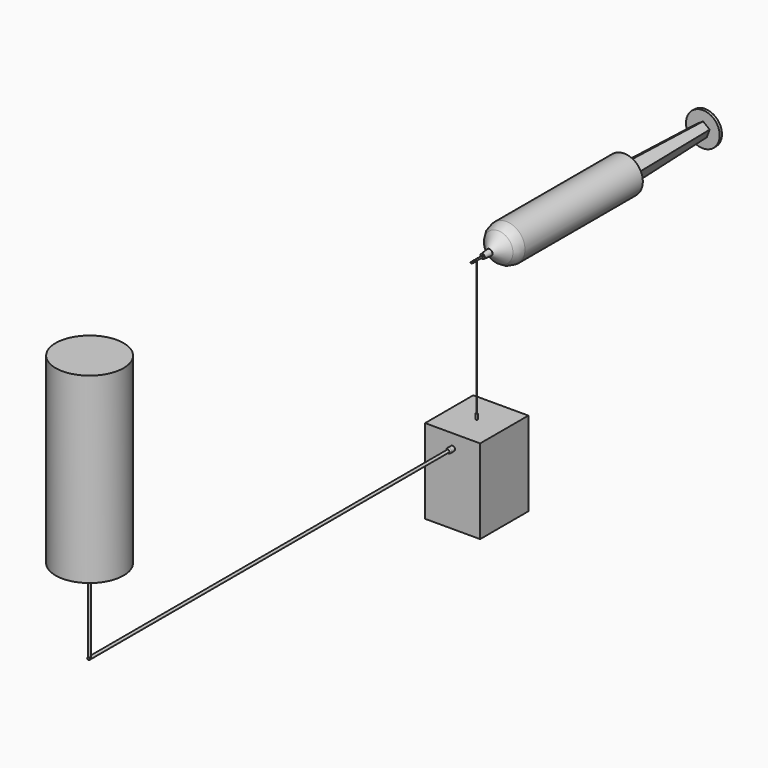
from build123d import *

# Parameters (mm, degrees)
F0_R         = 6.635
F1_DEPTH     = 60
F2_R         = 5.5640936577
F3_DEPTH     = 55
F5_DEPTH     = 90
F5_TAPER     = 1.5
F6_R         = 6
F7_DEPTH     = 1
F8_SIZE      = 5.5
F9_R         = 5
F10_R        = 1.1188654797
F11_DEPTH    = 3
F11_TAPER    = 6
F12_R        = 0.2661166515
F13_DEPTH    = 5
F15_START    = -0.7
F14_R        = 0.3090418991
F14_R_2      = 0.2661166515
F15_DEPTH    = 0.76
F17_START    = -2
F16_R        = 0.3072145748
F17_DEPTH    = 0.79
F19_R        = 0.1295808952
F20_DEPTH    = 50
F21_W        = 19.5904374123
F21_H        = 21.4598029852
F22_DEPTH    = 30
F23_R        = 0.3370193149
F24_DEPTH    = 2
F25_R        = 0.3
F26_R        = 0.8572593425
F27_DEPTH    = 2
F28_R        = 0.4
F29_R        = 1.2929704819
F29_R_2      = 1.8897224416
F29_R_3      = 1.1340105919
F30_DEPTH    = 1
F31_R        = 0.4652474762
F32_DEPTH    = 160
F35_R        = 0.4356898576
F36_DEPTH    = 30
F37_F1_R     = 0.02
F37_F2_R     = 0.02
F37_T6_ANGLE = 55.0572993012
F37_S7_R     = 0.4652474762
F37_T8_DEPTH = 2
F38_R        = 12.0941748202
F39_DEPTH    = 65


# Not quite as in the source:
# - a fillet or chamfer that OpenCascade refuses, or shapes differently, is made with other operations: its cross-section is extruded or revolved along the edge and cut away or added
# - a feature of the source that left no trace in its solid (it failed there, or was rolled back) is left out


with BuildPart() as f1:
    # F0 (on Front) → F1 (new body)
    with BuildSketch(Plane.XZ):
        Circle(F0_R)
    extrude(amount=F1_DEPTH)

    # F2 (on face) → F3 (cut)
    with BuildSketch(Plane(origin=(0, 0, 0), x_dir=(-1, 0, 0), z_dir=(0, 1, 0))):
        Circle(F2_R)
    extrude(amount=-F3_DEPTH, mode=Mode.SUBTRACT)

    # F4 (on face) → F5 (join)
    with BuildSketch(Plane(origin=(0, -55, 0), x_dir=(-1, 0, 0), z_dir=(0, 1, 0))):
        Polygon((-0.2330018257, 5.4173569127), (-5.2242141168, 1.452457446), (-2.995740063, -4.5196888438), (3.3727449364, -4.24577877), (5.080211069, 1.8956532552), align=None)
    extrude(amount=F5_DEPTH, taper=F5_TAPER)

    # F6 (on face) → F7 (join)
    with BuildSketch(Plane(origin=(0, 35, 0), x_dir=(-1, 0, 0), z_dir=(0, 1, 0))):
        Circle(F6_R)
    extrude(amount=F7_DEPTH)

    # F8
    f8_edges = [f1.edges().sort_by_distance(p)[0] for p in [
        (-6.635, -60, 0),
    ]]
    chamfer(f8_edges, length=F8_SIZE)

    # F9
    f9_edges = [f1.edges().sort_by_distance(p)[0] for p in [
        (-6.635, -54.5, 0),
    ]]
    fillet(f9_edges, radius=F9_R)

    # F10 (on face) → F11 (join)
    with BuildSketch(Plane.XZ.offset(60)):
        Circle(F10_R)
    extrude(amount=F11_DEPTH, taper=F11_TAPER)


with BuildPart() as f13:
    # F12 (on face) → F13 (new body)
    with BuildSketch(Plane.XZ.offset(63)):
        Circle(F12_R)
    extrude(amount=F13_DEPTH)


with BuildPart() as f15:
    # F14 (on face) → F15 (new body)
    with BuildSketch(Plane.XZ.offset(68).offset(F15_START)):
        Circle(F14_R)
        Circle(F14_R_2, mode=Mode.SUBTRACT)
    extrude(amount=-F15_DEPTH)


with BuildPart() as f17:
    # F16 (on face) → F17 (new body)
    with BuildSketch(Plane.XZ.offset(68).offset(F17_START)):
        Circle(F16_R)
    extrude(amount=-F17_DEPTH)


with BuildPart() as f20:
    # F19 (on Top) → F20 (new body)
    with BuildSketch(Plane.XY):
        with Locations((0, -65.6076744199)):
            Circle(F19_R)
    extrude(amount=-F20_DEPTH)


with BuildPart() as f22:
    # F21 (on face) → F22 (new body)
    with BuildSketch(Plane(origin=(0, 0, -50), x_dir=(1, 0, 0), z_dir=(0, 0, -1))):
        with Locations((0, 65.6076744199)):
            Rectangle(F21_W, F21_H)
    extrude(amount=F22_DEPTH)

    # F29 (on face) → F30 (cut)
    with BuildSketch(Plane(origin=(-9.7952187061, 0, 0), x_dir=(0, -1, 0), z_dir=(-1, 0, 0))):
        with Locations((59.0209439397, -53.7652634084)):
            Circle(F29_R)
        with Locations((59.1616034508, -58.758571744)):
            Circle(F29_R_2)
        with Locations((59.3022592366, -63.3299127221)):
            Circle(F29_R_3)
    extrude(amount=-F30_DEPTH, mode=Mode.SUBTRACT)


with BuildPart() as f24:
    # F23 (on face) → F24 (new body)
    with BuildSketch(Plane.XY.offset(-50)):
        with Locations((0, -65.6058713794)):
            Circle(F23_R)
    extrude(amount=F24_DEPTH)

    # F25
    f25_edges = [f24.edges().sort_by_distance(p)[0] for p in [
        (-0.337019, -65.605871, -48),
    ]]
    fillet(f25_edges, radius=F25_R)


with BuildPart() as f27:
    # F26 (on face) → F27 (new body)
    with BuildSketch(Plane.XZ.offset(76.3375759125)):
        with Locations((0, -54.7743812203)):
            Circle(F26_R)
    extrude(amount=F27_DEPTH)

    # F28
    f28_edges = [f27.edges().sort_by_distance(p)[0] for p in [
        (-0.857259, -78.337576, -54.774381),
    ]]
    fillet(f28_edges, radius=F28_R)


with BuildPart() as f32:
    # F31 (on face) → F32 (new body)
    with BuildSketch(Plane.XZ.offset(78.3375759125)):
        with Locations((0, -54.7743812203)):
            Circle(F31_R)
    extrude(amount=F32_DEPTH)

    # F35 (on offset) → F36 (join)
    with BuildSketch(Plane.XY.offset(-55)):
        with Locations((0, -237.8518730402)):
            Circle(F35_R)
    extrude(amount=F36_DEPTH)

    # F37: fillet of radius 0.02 on 3 edges, made by hand

    # F37_f1
    f37_f1_edges = [f32.edges().sort_by_distance(p)[0] for p in [
        (-0.4652474762, -238.3375759125, -54.7743812203),
    ]]
    fillet(f37_f1_edges, radius=F37_F1_R)

    # F37_f2
    f37_f2_edges = [f32.edges().sort_by_distance(p)[0] for p in [
        (-0.4356898576, -237.8518730402, -55),
    ]]
    fillet(f37_f2_edges, radius=F37_F2_R)


with BuildPart() as f37_tool4:
    # F37_s5 → F37_t6 (revolve)
    with BuildSketch(Plane(origin=(-97.4865926005, -187.0415928726, 0), x_dir=(0, 0, 1), z_dir=(-0.4621920882, -0.8867798338, 0))):
        with BuildLine():
            ThreePointArc((-54.98, -110.3689437327), (-54.9941421356, -110.3630858683), (-55, -110.3489437327))
            Line((-55, -110.3489437327), (-55.0004, -110.3489437327))
            Line((-55.0004, -110.3489437327), (-55.0004, -110.3693437327))
            Line((-55.0004, -110.3693437327), (-54.98, -110.3693437327))
            Line((-54.98, -110.3693437327), (-54.98, -110.3689437327))
        make_face()
    revolve(axis=Axis((0, -237.8518730402, -55), (0, 0, 1)), revolution_arc=F37_T6_ANGLE)

    # F37_s7 → F37_t8 (cut, symmetric)
    with BuildSketch(Plane.XZ.offset(237.9)):
        with Locations((0, -54.7743812203)):
            Circle(F37_S7_R)
    extrude(amount=F37_T8_DEPTH, both=True, mode=Mode.SUBTRACT)


with BuildPart() as f32_1:
    add(f32.part)

    # F37_t3: cut F37_tool4
    add(f37_tool4.part, mode=Mode.SUBTRACT)

    # F38 (on face) → F39 (join)
    with BuildSketch(Plane.XY.offset(-25)):
        with Locations((0, -237.8518730402)):
            Circle(F38_R)
    extrude(amount=F39_DEPTH)


solid = Compound([f1.part, f13.part, f15.part, f17.part, f20.part, f22.part, f24.part, f27.part, f32_1.part])
